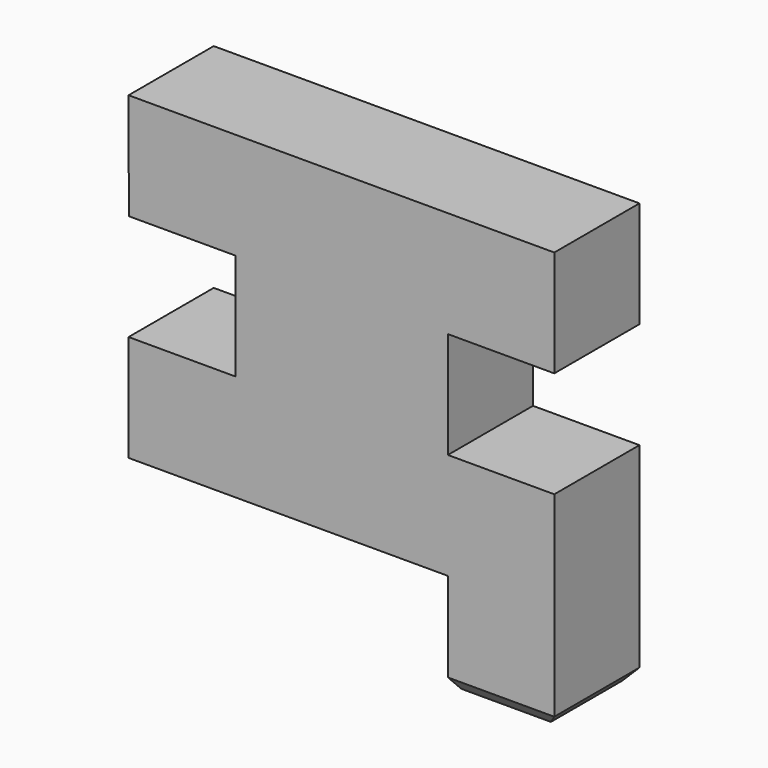
from build123d import *

# Parameters (mm, degrees)
F1_DEPTH = 6.35
F2_SIZE  = 1.016
F3_SIZE  = 1.016


# Not quite as in the source:
# - a feature of the source that left no trace in its solid (it failed there, or was rolled back) is left out


with BuildPart() as f1:
    # F0 (on Front) → F1 (new body)
    with BuildSketch(Plane.XZ):
        Polygon((25.4, 0), (0, 0), (0.0169261405, -6.35), (6.3669261405, -6.35), (6.3669261405, -12.7), (0, -12.7), (0, -19.05), (19.05, -19.05), (19.05, -25.4), (25.4, -25.4), (25.4, -12.7), (19.05, -12.7), (19.05, -6.35), (25.4, -6.35), align=None)
    extrude(amount=F1_DEPTH)

    # F2
    f2_edges = [f1.edges().sort_by_distance(p)[0] for p in [
        (22.225, -6.35, -25.4),
    ]]
    chamfer(f2_edges, length=F2_SIZE)

    # F3
    f3_edges = [f1.edges().sort_by_distance(p)[0] for p in [
        (25.4, -2.667, -25.4),
    ]]
    chamfer(f3_edges, length=F3_SIZE)


solid = f1.part
